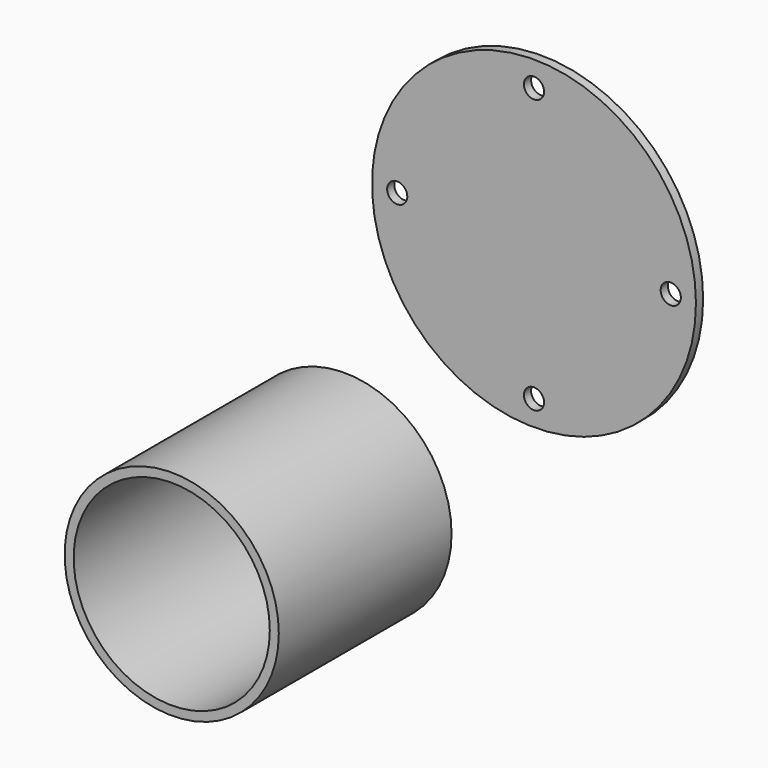
from build123d import *

# Parameters (mm, degrees)
F0_R     = 57.15
F0_R_2   = 3.556
F1_DEPTH = 3.175
F2_R     = 37.7825
F2_R_2   = 34.6075
F3_DEPTH = 76.2


# Not quite as in the source:
# - a feature names something its author has since deleted; it is built from what else it names


with BuildPart() as f1:
    # F0 (on Front) → F1 (new body)
    with BuildSketch(Plane.XZ):
        Circle(F0_R)
        with Locations((0, -48.26)):
            Circle(F0_R_2, mode=Mode.SUBTRACT)
        with Locations((-48.26, 0)):
            Circle(F0_R_2, mode=Mode.SUBTRACT)
        with Locations((48.26, 0)):
            Circle(F0_R_2, mode=Mode.SUBTRACT)
        with Locations((0, 48.26)):
            Circle(F0_R_2, mode=Mode.SUBTRACT)
    extrude(amount=F1_DEPTH)


with BuildPart() as f3:
    # F2 (on Front) → F3 (new body)
    with BuildSketch(Plane.XZ):
        with Locations((-69.4049596786, -101.8172428012)):
            Circle(F2_R)
        with Locations((-69.4049596786, -101.8172428012)):
            Circle(F2_R_2, mode=Mode.SUBTRACT)
    extrude(amount=F3_DEPTH)


solid = Compound([f1.part, f3.part])
